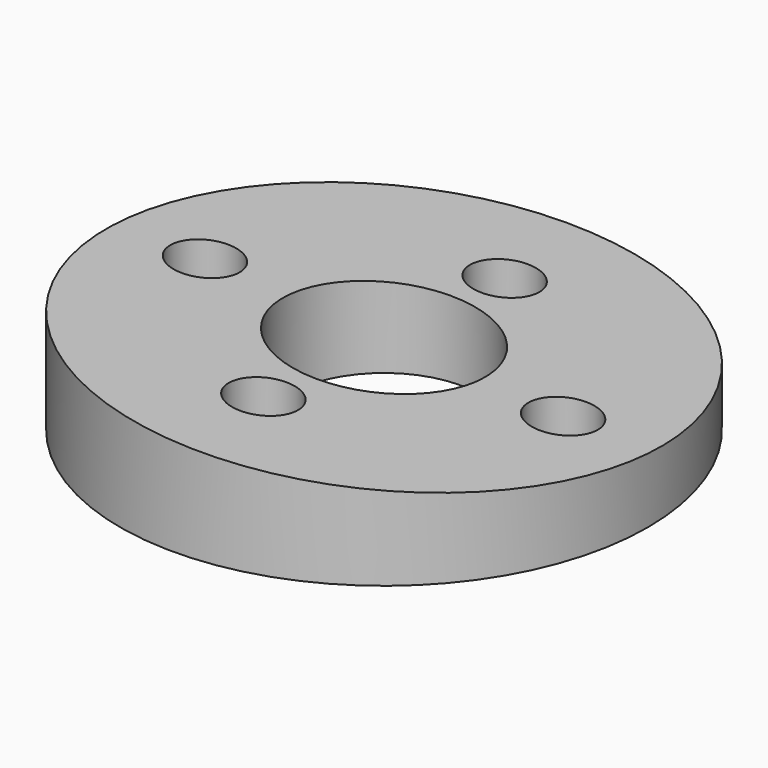
from build123d import *

# Parameters (mm, degrees)
F0_R     = 14
F0_R_2   = 1.75
F0_R_3   = 5.1
F1_DEPTH = 10
F5_W     = 30
F5_H     = 3
F6_DEPTH = 40


with BuildPart() as f1:
    # F0 (on Top) → F1 (new body)
    with BuildSketch(Plane.XY):
        Circle(F0_R)
        with Locations((0, -8)):
            Circle(F0_R_2, mode=Mode.SUBTRACT)
        with Locations((-9.5, 0)):
            Circle(F0_R_2, mode=Mode.SUBTRACT)
        Circle(F0_R_3, mode=Mode.SUBTRACT)
        with Locations((9.5, 0)):
            Circle(F0_R_2, mode=Mode.SUBTRACT)
        with Locations((0, 8)):
            Circle(F0_R_2, mode=Mode.SUBTRACT)
    extrude(amount=F1_DEPTH)

    # F5 (on face) → F6 (intersect)
    with BuildSketch(Plane(origin=(17.6776695297, -17.6776695297, 0), x_dir=(0.7071067812, 0.7071067812, 0), z_dir=(0.7071067812, -0.7071067812, 0))):
        Polygon((-15, 5.6246599058), (-15, 0), (15, 0), (15, 3), align=None)
        with Locations((0, -1.5)):
            Rectangle(F5_W, F5_H)
    extrude(amount=-F6_DEPTH, mode=Mode.INTERSECT)


solid = f1.part
